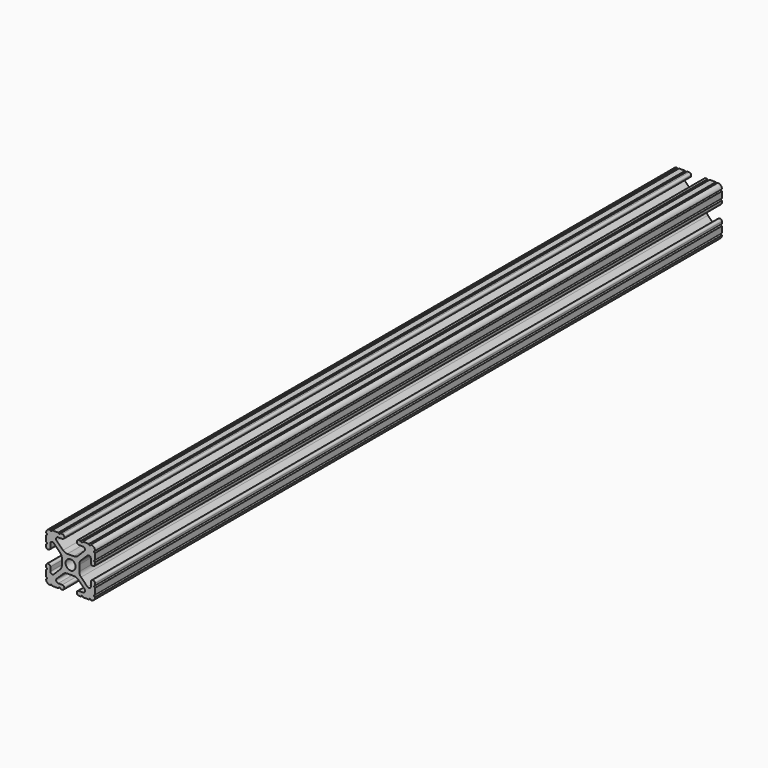
from build123d import *

# Parameters (mm, degrees)
F0_R     = 2.6035
F1_DEPTH = 406.4


# Not quite as in the source:
# - ends of sketch curves that miss each other by under 0.0002 mm in the source are joined


with BuildPart() as f1:
    # F0 (on Front) → F1 (new body)
    with BuildSketch(Plane.XZ):
        with BuildLine():
            ThreePointArc((-3.9522606035, -5.4236922052), (-2.9229262099, -4.7369294977), (-1.7092422, -4.4958))
            Line((-1.7092422, -4.4958), (1.7092422, -4.4958))
            ThreePointArc((1.7092422, -4.4958), (2.9229262099, -4.7369294977), (3.9522606035, -5.4236922052))
            Line((3.9522606035, -5.4236922052), (7.1796402, -8.6451948))
            ThreePointArc((7.1796402, -8.6451948), (7.4147391594, -9.822808991), (6.416421, -10.4902))
            Line((6.416421, -10.4902), (4.28752, -10.4902))
            ThreePointArc((4.28752, -10.4902), (3.5457508444, -10.7974508444), (3.2385, -11.53922))
            Line((3.2385, -11.53922), (3.2385, -11.65098))
            ThreePointArc((3.2385, -11.65098), (3.5457508444, -12.3927491556), (4.28752, -12.7))
            Line((4.28752, -12.7), (5.3171344, -12.7))
            ThreePointArc((5.3171344, -12.7), (5.8251344, -12.192), (6.3331344, -12.7))
            Line((6.3331344, -12.7), (9.5504508, -12.7))
            ThreePointArc((9.5504508, -12.7), (10.0583746, -12.1920000057), (10.5664507771, -12.6998476))
            ThreePointArc((10.5664507771, -12.6998476), (12.0825404752, -12.0825045568), (12.6998469825, -10.5664000074))
            ThreePointArc((12.6998469825, -10.5664000074), (12.1920000057, -10.0583238), (12.7, -9.5504))
            Line((12.7, -9.5504), (12.7, -6.3330836))
            ThreePointArc((12.7, -6.3330836), (12.192, -5.8250836), (12.7, -5.3170836))
            Line((12.7, -5.3170836), (12.7, -4.2874692))
            ThreePointArc((12.7, -4.2874692), (12.3927491556, -3.5457000444), (11.65098, -3.2384492))
            Line((11.65098, -3.2384492), (11.53922, -3.2384492))
            ThreePointArc((11.53922, -3.2384492), (10.7974508444, -3.5457000444), (10.4902, -4.2874692))
            Line((10.4902, -4.2874692), (10.4902, -6.4020954))
            ThreePointArc((10.4902, -6.4020954), (9.8565053438, -7.3510699477), (8.7371366164, -7.1294051977))
            Line((8.7371366164, -7.1294051977), (5.4410102, -3.8408102))
            ThreePointArc((5.4410102, -3.8408102), (4.7508771577, -2.8098852335), (4.5085, -1.5931896))
            Line((4.5085, -1.5931896), (4.5085, 1.5931896))
            ThreePointArc((4.5085, 1.5931896), (4.7508771577, 2.8098852335), (5.4410028439, 3.840817573))
            Line((5.4410028439, 3.840817573), (8.7371428, 7.129399))
            ThreePointArc((8.7371428, 7.129399), (9.8565053438, 7.3510699477), (10.4902, 6.4020954))
            Line((10.4902, 6.4020954), (10.4902, 4.2874692))
            ThreePointArc((10.4902, 4.2874692), (10.7974508444, 3.5457000444), (11.53922, 3.2384492))
            Line((11.53922, 3.2384492), (11.65098, 3.2384492))
            ThreePointArc((11.65098, 3.2384492), (12.3927491556, 3.5457000444), (12.7, 4.2874692))
            Line((12.7, 4.2874692), (12.7, 5.3170836))
            ThreePointArc((12.7, 5.3170836), (12.192, 5.8250836), (12.7, 6.3330836))
            Line((12.7, 6.3330836), (12.7, 9.5504))
            ThreePointArc((12.7, 9.5504), (12.1920000057, 10.0583238), (12.6998476, 10.5663999771))
            ThreePointArc((12.6998476, 10.5663999771), (12.0825404752, 12.0825045568), (10.5664508001, 12.6998475939))
            ThreePointArc((10.5664508001, 12.6998475939), (10.0583746, 12.1920000057), (9.5504508, 12.7))
            Line((9.5504508, 12.7), (6.3331344, 12.7))
            ThreePointArc((6.3331344, 12.7), (5.8251344, 12.192), (5.3171344, 12.7))
            Line((5.3171344, 12.7), (4.28752, 12.7))
            ThreePointArc((4.28752, 12.7), (3.5457508444, 12.3927491556), (3.2385, 11.65098))
            Line((3.2385, 11.65098), (3.2385, 11.53922))
            ThreePointArc((3.2385, 11.53922), (3.5457508444, 10.7974508444), (4.28752, 10.4902))
            Line((4.28752, 10.4902), (6.4767968, 10.4902))
            ThreePointArc((6.4767968, 10.4902), (7.4322289723, 9.8514044384), (7.2070407772, 8.7243726366))
            Line((7.2070407772, 8.7243726366), (3.898265, 5.4231794))
            ThreePointArc((3.898265, 5.4231794), (2.8691189654, 4.7367887684), (1.6557752, 4.4958))
            Line((1.6557752, 4.4958), (-1.6557752, 4.4958))
            ThreePointArc((-1.6557752, 4.4958), (-2.8691189654, 4.7367887684), (-3.8982723561, 5.423172027))
            Line((-3.8982723561, 5.423172027), (-7.2070468, 8.7243666))
            ThreePointArc((-7.2070468, 8.7243666), (-7.4322289723, 9.8514044384), (-6.4767968, 10.4902))
            Line((-6.4767968, 10.4902), (-4.28752, 10.4902))
            ThreePointArc((-4.28752, 10.4902), (-3.5457508444, 10.7974508444), (-3.2385, 11.53922))
            Line((-3.2385, 11.53922), (-3.2385, 11.65098))
            ThreePointArc((-3.2385, 11.65098), (-3.5457508444, 12.3927491556), (-4.28752, 12.7))
            Line((-4.28752, 12.7), (-5.3171344, 12.7))
            ThreePointArc((-5.3171344, 12.7), (-5.8251344, 12.192), (-6.3331344, 12.7))
            Line((-6.3331344, 12.7), (-9.5504508, 12.7))
            ThreePointArc((-9.5504508, 12.7), (-10.0583746, 12.1920000057), (-10.5664507771, 12.6998476))
            ThreePointArc((-10.5664507771, 12.6998476), (-12.0825404752, 12.0825045568), (-12.6998469825, 10.5664000074))
            ThreePointArc((-12.6998469825, 10.5664000074), (-12.1920000057, 10.0583238), (-12.7, 9.5504))
            Line((-12.7, 9.5504), (-12.7, 6.3330836))
            ThreePointArc((-12.7, 6.3330836), (-12.192, 5.8250836), (-12.7, 5.3170836))
            Line((-12.7, 5.3170836), (-12.7, 4.2874692))
            ThreePointArc((-12.7, 4.2874692), (-12.3927491556, 3.5457000444), (-11.65098, 3.2384492))
            Line((-11.65098, 3.2384492), (-11.53922, 3.2384492))
            ThreePointArc((-11.53922, 3.2384492), (-10.7974508444, 3.5457000444), (-10.4902, 4.2874692))
            Line((-10.4902, 4.2874692), (-10.4902, 6.4020954))
            ThreePointArc((-10.4902, 6.4020954), (-9.8565053438, 7.3510699477), (-8.7371366164, 7.1294051977))
            Line((-8.7371366164, 7.1294051977), (-5.4410102, 3.8408102))
            ThreePointArc((-5.4410102, 3.8408102), (-4.7508771577, 2.8098852335), (-4.5085, 1.5931896))
            Line((-4.5085, 1.5931896), (-4.5085, -1.5931896))
            ThreePointArc((-4.5085, -1.5931896), (-4.7508771577, -2.8098852335), (-5.4410028439, -3.840817573))
            Line((-5.4410028439, -3.840817573), (-8.7371428, -7.129399))
            ThreePointArc((-8.7371428, -7.129399), (-9.8565053438, -7.3510699477), (-10.4902, -6.4020954))
            Line((-10.4902, -6.4020954), (-10.4902, -4.2874692))
            ThreePointArc((-10.4902, -4.2874692), (-10.7974508444, -3.5457000444), (-11.53922, -3.2384492))
            Line((-11.53922, -3.2384492), (-11.65098, -3.2384492))
            ThreePointArc((-11.65098, -3.2384492), (-12.3927491556, -3.5457000444), (-12.7, -4.2874692))
            Line((-12.7, -4.2874692), (-12.7, -5.3170836))
            ThreePointArc((-12.7, -5.3170836), (-12.192, -5.8250836), (-12.7, -6.3330836))
            Line((-12.7, -6.3330836), (-12.7, -9.5504))
            ThreePointArc((-12.7, -9.5504), (-12.1920000057, -10.0583238), (-12.6998476, -10.5663999771))
            ThreePointArc((-12.6998476, -10.5663999771), (-12.0825404752, -12.0825045568), (-10.5664508001, -12.6998475939))
            ThreePointArc((-10.5664508001, -12.6998475939), (-10.0583746, -12.1920000057), (-9.5504508, -12.7))
            Line((-9.5504508, -12.7), (-6.3331344, -12.7))
            ThreePointArc((-6.3331344, -12.7), (-5.8251344, -12.192), (-5.3171344, -12.7))
            Line((-5.3171344, -12.7), (-4.28752, -12.7))
            ThreePointArc((-4.28752, -12.7), (-3.5457508444, -12.3927491556), (-3.2385, -11.65098))
            Line((-3.2385, -11.65098), (-3.2385, -11.53922))
            ThreePointArc((-3.2385, -11.53922), (-3.5457508444, -10.7974508444), (-4.28752, -10.4902))
            Line((-4.28752, -10.4902), (-6.416421, -10.4902))
            ThreePointArc((-6.416421, -10.4902), (-7.4147391594, -9.822808991), (-7.1796418951, -8.6451931018))
            Line((-7.1796418951, -8.6451931018), (-3.9522606035, -5.4236922052))
        make_face()
        Circle(F0_R, mode=Mode.SUBTRACT)
    extrude(amount=F1_DEPTH)


solid = f1.part
